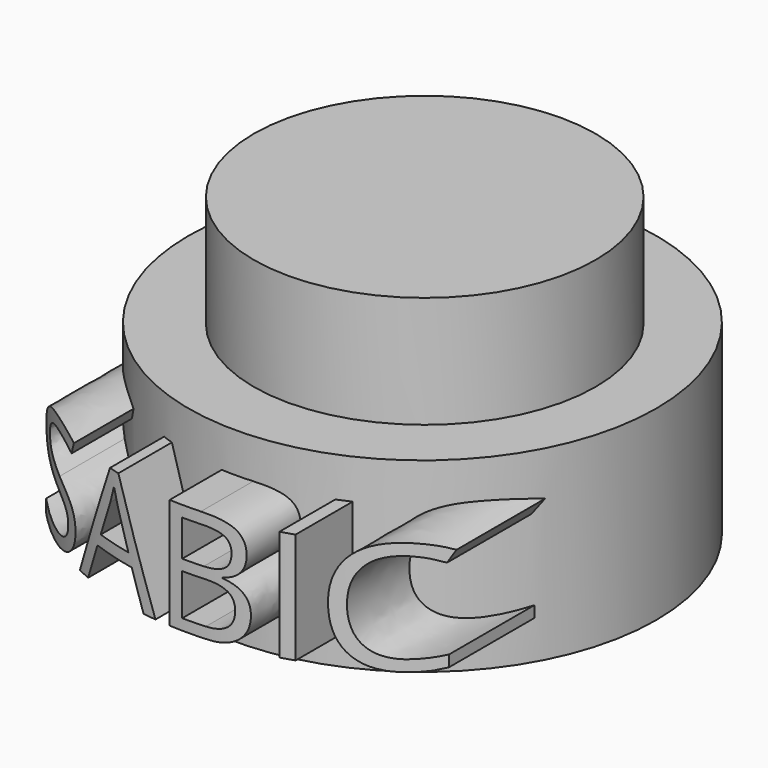
from build123d import *

# Parameters (mm, degrees)
F0_R         = 31.394129746
F1_DEPTH     = 25
F2_R         = 22.9407724692
F3_DEPTH     = 15
F6_TEXT_SIZE = 20.8333333333
F7_DEPTH     = 50
F8_R         = 40
F9_DEPTH     = 65


# Not quite as in the source:
# - the program builds the solid bodies; features that only make, move or delete a surface that nothing else refers to are left out
# - Text() gives the source's letters only with a copy of the font that has no kerning and outlines rounded to 1/6400 em; it was checked with that copy


with BuildPart() as f1:
    # F0 (on Top) → F1 (new body)
    with BuildSketch(Plane.XY):
        with Locations((-0.4249103367, 0.1416336745)):
            Circle(F0_R)
    extrude(amount=F1_DEPTH)

    # F2 (on face) → F3 (join)
    with BuildSketch(Plane.XY.offset(25)):
        Circle(F2_R)
    extrude(amount=F3_DEPTH)

    # F6 (on Front) → F7 (join)
    with BuildSketch(Plane.XZ):
        with Locations((-28.9457017146, 4.811364842)):
            Text('SABIC', F6_TEXT_SIZE, font='Open Sans', text_align=(TextAlign.LEFT, TextAlign.BOTTOM))
    extrude(amount=F7_DEPTH)

    # F8 (on Top) → F9 (intersect)
    with BuildSketch(Plane.XY):
        Circle(F8_R)
    extrude(amount=F9_DEPTH, mode=Mode.INTERSECT)


solid = f1.part
